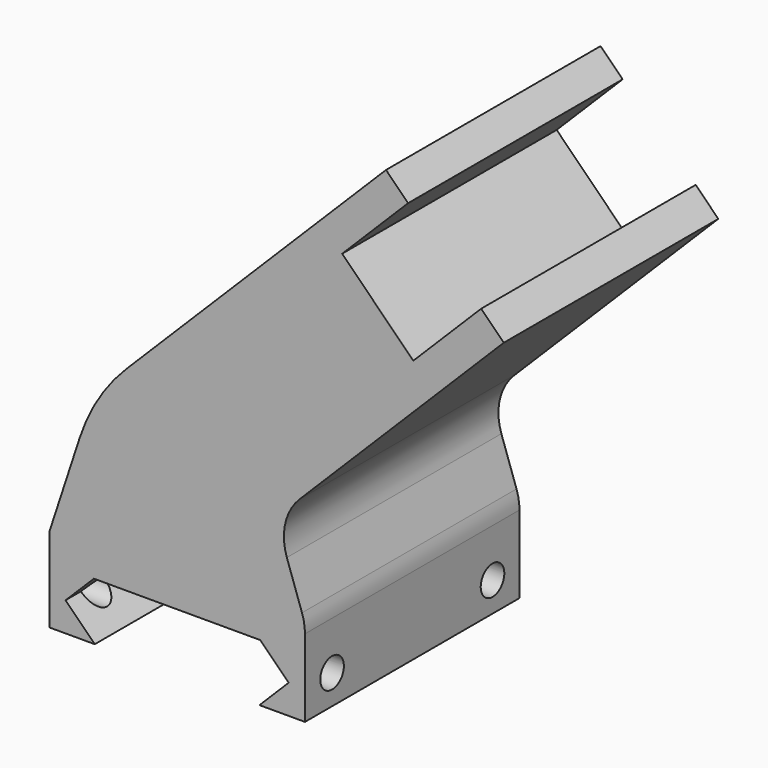
from build123d import *

# Parameters (mm, degrees)
F1_DEPTH = 25.4
F3_D     = 2.794
F3_DEPTH = 25.4
F3_TIP   = 0.8394022848
F4_D     = 2.794
F4_DEPTH = 25.4
F4_START = 10.1278152
F4_TIP   = 0.8394022848
F5_R     = 18.0883597705
F6_R     = 5.08


# Not quite as in the source:
# - ends of sketch curves that miss each other by under 0.0002 mm in the source are joined
# - a feature names something its author has since deleted; it is built from what else it names


with BuildPart() as f1:
    # F0 (on Front) → F1 (new body)
    with BuildSketch(Plane.XZ):
        Polygon((11.0066256276, -6.5430273301), (8.240193387, -9.310965985), (12.5485987193, -9.310965985), (12.5485987193, -1.1086727812), (9.7906497979, 6.8444932552), (24.9488617122, 22.0027051695), (31.3820510637, 28.435894521), (29.2404852808, 30.5774603039), (22.8072959293, 24.1442709524), (16.0729033236, 30.8786635582), (22.3196721338, 37.1254323684), (20.2273843878, 39.2177201144), (14.0302290969, 33.0205648235), (13.9806155776, 32.9709513042), (-7.4406042695, 11.5497314571), (-11.6305711889, -1.2286720797), (-11.6305711889, -9.3063699081), (-7.3613829189, -9.3063699081), (-10.1278151595, -6.5384312532), (-7.4425795762, -3.8636476732), (8.3167760077, -3.8636476732), align=None)
    extrude(amount=F1_DEPTH)

    # F3 (one way)
    with BuildSketch(Plane(origin=(0, 0, 0), x_dir=(0, 1, 0), z_dir=(-1, 0, 0))):
        with Locations((-22.1899207681, 6.5197679214), (-3.1917574815, 6.5197679214)):
            Circle(F3_D / 2)
    extrude(amount=-F3_DEPTH, mode=Mode.SUBTRACT)
    with Locations(Plane(origin=(0, 0, 0), x_dir=(0, 1, 0), z_dir=(-1, 0, 0))):
        with Locations((-22.1899207681, 6.5197679214), (-3.1917574815, 6.5197679214)):
            with Locations((0, 0, -(F3_DEPTH + F3_TIP / 2))):  # 118° drill point
                Cone(0, F3_D / 2, F3_TIP, mode=Mode.SUBTRACT)

    # F4
    # its depths count from where the whole tool has entered the part; down to there all is cleared
    with Locations(Plane.YZ.offset(-F4_START)):
        with Locations((-3.1917574815, -6.5197679214), (-22.1899207681, -6.5197679214)):
            Hole(F4_D / 2, depth=F4_DEPTH)
            with Locations((0, 0, -(F4_DEPTH + F4_TIP / 2))):  # 118° drill point
                Cone(0, F4_D / 2, F4_TIP, mode=Mode.SUBTRACT)

    # F5
    f5_edges = [f1.edges().sort_by_distance(p)[0] for p in [
        (-7.440604, -12.7, 11.549731),
    ]]
    fillet(f5_edges, radius=F5_R)

    # F6
    f6_edges = [f1.edges().sort_by_distance(p)[0] for p in [
        (9.79065, -12.7, 6.844493),
        (12.548599, -12.7, -1.108673),
    ]]
    fillet(f6_edges, radius=F6_R)


solid = f1.part
